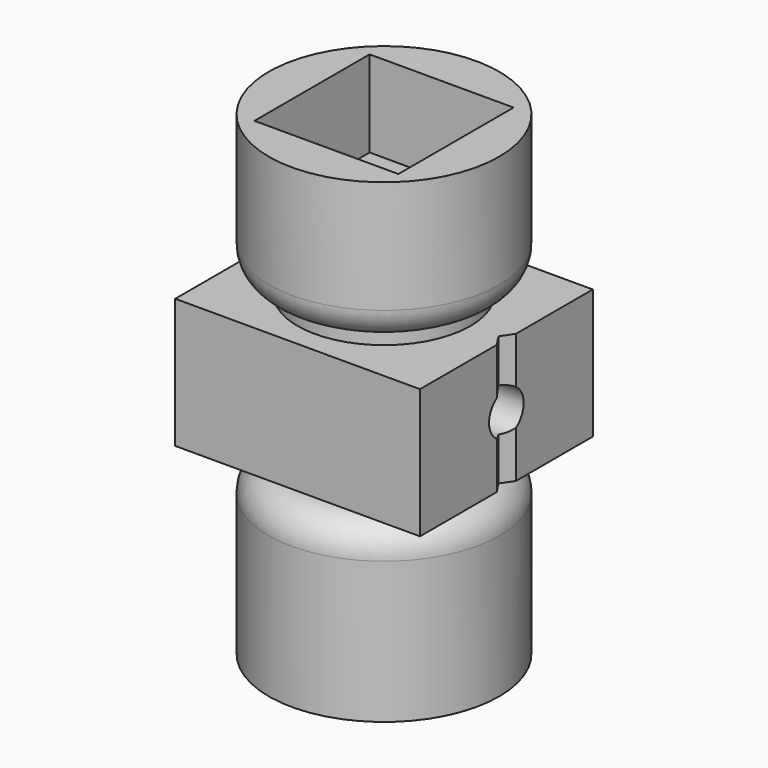
from build123d import *

# Parameters (mm, degrees)
F0_W      = 17
F0_H      = 15
F1_DEPTH  = 4.5
F2_R      = 6
F3_DEPTH  = 1
F4_R      = 6
F5_DEPTH  = 1
F6_R      = 1.5
F7_DEPTH  = 17.001
F9_DEPTH  = 10.001
F10_R     = 8
F11_DEPTH = 10
F12_R     = 8
F12_R_2   = 6
F13_DEPTH = 12
F16_DEPTH = 6
F17_W     = 10
F17_H     = 10
F18_DEPTH = 6


# Not quite as in the source:
# - a fillet or chamfer that OpenCascade refuses, or shapes differently, is made with other operations: its cross-section is extruded or revolved along the edge and cut away or added


with BuildPart() as f1:
    # F0 (on Top) → F1 (new body, symmetric)
    with BuildSketch(Plane.XY):
        Rectangle(F0_W, F0_H)
    extrude(amount=F1_DEPTH, both=True)

    # F2 (on face) → F3 (join)
    with BuildSketch(Plane.XY.offset(4.5)):
        Circle(F2_R)
    extrude(amount=F3_DEPTH)

    # F4 (on face) → F5 (join)
    with BuildSketch(Plane(origin=(0, 0, -4.5), x_dir=(1, 0, 0), z_dir=(0, 0, -1))):
        Circle(F4_R)
    extrude(amount=F5_DEPTH)

    # F6 (on face) → F7 (cut, through all)
    with BuildSketch(Plane.YZ.offset(8.5)):
        Circle(F6_R)
    extrude(amount=-F7_DEPTH, mode=Mode.SUBTRACT)

    # F8 (on face) → F9 (cut, through all)
    with BuildSketch(Plane(origin=(0, 0, -4.5), x_dir=(1, 0, 0), z_dir=(0, 0, -1))):
        Polygon((8.5, 0.8288529099), (7.9405334204, 0), (8.5, -0.8288529099), align=None)
        Polygon((-8.5, -0.7952927344), (-7.8937744095, 0), (-8.5, 0.7952927344), align=None)
    extrude(amount=-F9_DEPTH, mode=Mode.SUBTRACT)

    # F10 (on face) → F11 (join)
    with BuildSketch(Plane.XY.offset(5.5)):
        Circle(F10_R)
    extrude(amount=F11_DEPTH)

    # F14: fillet of radius 2.1727922061 on 1 edges, made by hand

    # F14_s1 → F14_t2 (revolve, cut)
    with BuildSketch(Plane.XZ):
        with BuildLine():
            ThreePointArc((8, 7.6659106225), (7.4235266107, 6.1918712044), (6, 5.5))
            Line((6, 5.5), (8, 5.5))
            Line((8, 5.5), (8, 7.6659106225))
        make_face()
    revolve(axis=Axis((0, 0, 5.5), (0, 0, 1)), mode=Mode.SUBTRACT)

    # F17 (on face) → F18 (cut)
    with BuildSketch(Plane.XY.offset(15.5)):
        Rectangle(F17_W, F17_H)
    extrude(amount=-F18_DEPTH, mode=Mode.SUBTRACT)


with BuildPart() as f13:
    # F12 (on face) → F13 (new body)
    with BuildSketch(Plane(origin=(0, 0, -5.5), x_dir=(1, 0, 0), z_dir=(0, 0, -1))):
        Circle(F12_R)
        Circle(F12_R_2, mode=Mode.SUBTRACT)
        Circle(F12_R_2)
    extrude(amount=F13_DEPTH)

    # F14#2: fillet of radius 2.1727922061 on 1 edges, made by hand

    # F14_2_s1 → F14_2_t2 (revolve, cut)
    with BuildSketch(Plane.XZ):
        with BuildLine():
            ThreePointArc((8, -7.6727922061), (7.3636038969, -6.1363961031), (5.8272077939, -5.5))
            Line((5.8272077939, -5.5), (8, -5.5))
            Line((8, -5.5), (8, -7.6727922061))
        make_face()
    revolve(axis=Axis((0, 0, -5.5), (0, 0, -1)), mode=Mode.SUBTRACT)

    # F15 (on face) → F16 (cut)
    with BuildSketch(Plane(origin=(0, 0, -17.5), x_dir=(1, 0, 0), z_dir=(0, 0, -1))):
        Polygon((1.2821056222, 7.1357343822), (-1.2821056222, 7.1357343822), (-6.8207800608, -2.4575311519), (-5.6844085005, -4.5), (5.6844085005, -4.5), (6.8207800608, -2.4575311519), align=None)
    extrude(amount=-F16_DEPTH, mode=Mode.SUBTRACT)


solid = Compound([f1.part, f13.part])
